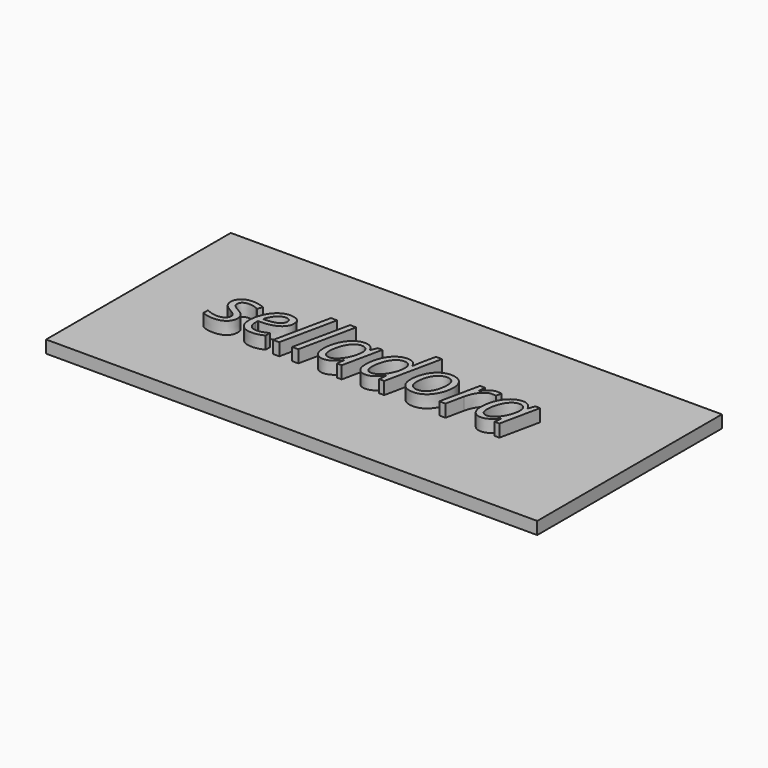
from build123d import *

# Parameters (mm, degrees)
F0_W         = 1000
F0_H         = 470
F1_DEPTH     = 25.4
F2_TEXT_SIZE = 152.9743584494
F3_DEPTH     = 25.4


# Not quite as in the source:
# - Text() gives the source's letters only with a copy of the font that has no kerning and outlines rounded to 1/6400 em; it was checked with that copy


with BuildPart() as f1:
    # F0 (on Top) → F1 (new body)
    with BuildSketch(Plane.XY):
        with Locations((10.936614126, 116.4468666955)):
            Rectangle(F0_W, F0_H)
    extrude(amount=F1_DEPTH)

    # F2 (on face) → F3 (join)
    with BuildSketch(Plane.XY.offset(25.4)):
        with Locations((-321.0719376802, 67.6936209202)):
            Text('selladora', F2_TEXT_SIZE, font='Open Sans', font_style=FontStyle.ITALIC, text_align=(TextAlign.LEFT, TextAlign.BOTTOM))
    extrude(amount=F3_DEPTH)


solid = f1.part
